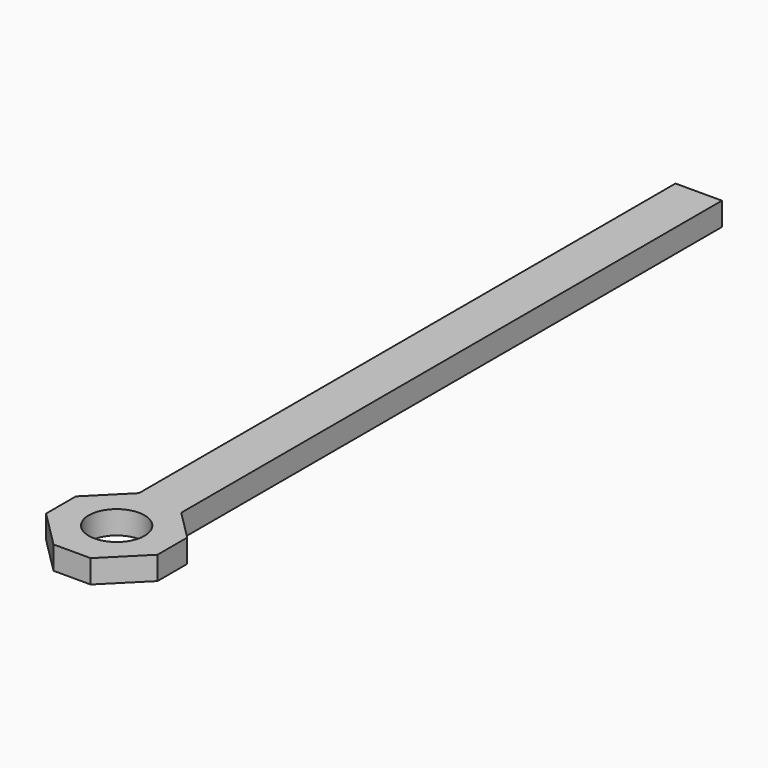
from build123d import *

# Parameters (mm, degrees)
F0_R         = 3
F0_W         = 5
F0_H         = 72
F1_DEPTH     = 2.5
F2_T1_DEPTH  = 23.0734639037
F2_T6_DEPTH  = 23.0734639037
F2_T11_DEPTH = 23.0734639037


# Not quite as in the source:
# - a fillet or chamfer that OpenCascade refuses, or shapes differently, is made with other operations: its cross-section is extruded or revolved along the edge and cut away or added


with BuildPart() as f1:
    # F0 (on Top) → F1 (new body)
    with BuildSketch(Plane.XY):
        Polygon((5, 6), (0, 6), (-3.7796038147, 6), (-3.7796038147, -6), (8.2203961853, -6), (8.2203961853, 6), align=None)
        with Locations((2.2203961853, 0)):
            Circle(F0_R, mode=Mode.SUBTRACT)
        with Locations((2.5, 42)):
            Rectangle(F0_W, F0_H)
    extrude(amount=F1_DEPTH)

    # F2: chamfer of 4 on 4 edges, made by hand

    # F2_s2 → F2_t1 (cut)
    with BuildSketch(Plane.XY.offset(-10.2867319519)):
        Polygon((4.2203961853, -6), (8.2203961853, -2), (8.2203961853, -6), align=None)
        Polygon((-3.7796038147, -2), (0.2203961853, -6), (-3.7796038147, -6), align=None)
    extrude(amount=F2_T1_DEPTH, mode=Mode.SUBTRACT)


with BuildPart() as f2_tool4:
    # F2_s5 → F2_t6 (new body)
    with BuildSketch(Plane.XY.offset(-10.2867319519)):
        Polygon((0.2203961853, 6), (-3.7796038147, 2), (-3.7796038147, 6), align=None)
    extrude(amount=F2_T6_DEPTH)

    split(bisect_by=Plane.YZ, keep=Keep.BOTTOM)


with BuildPart() as f1_1:
    add(f1.part)

    # F2_t3: cut F2_tool4
    add(f2_tool4.part, mode=Mode.SUBTRACT)


with BuildPart() as f2_tool9:
    # F2_s10 → F2_t11 (new body)
    with BuildSketch(Plane.XY.offset(-10.2867319519)):
        Polygon((4.2203961853, 6), (8.2203961853, 2), (8.2203961853, 6), align=None)
    extrude(amount=F2_T11_DEPTH)

    split(bisect_by=Plane.YZ.offset(5), keep=Keep.TOP)


with BuildPart() as f1_2:
    add(f1_1.part)

    # F2_t8: cut F2_tool9
    add(f2_tool9.part, mode=Mode.SUBTRACT)


solid = f1_2.part
